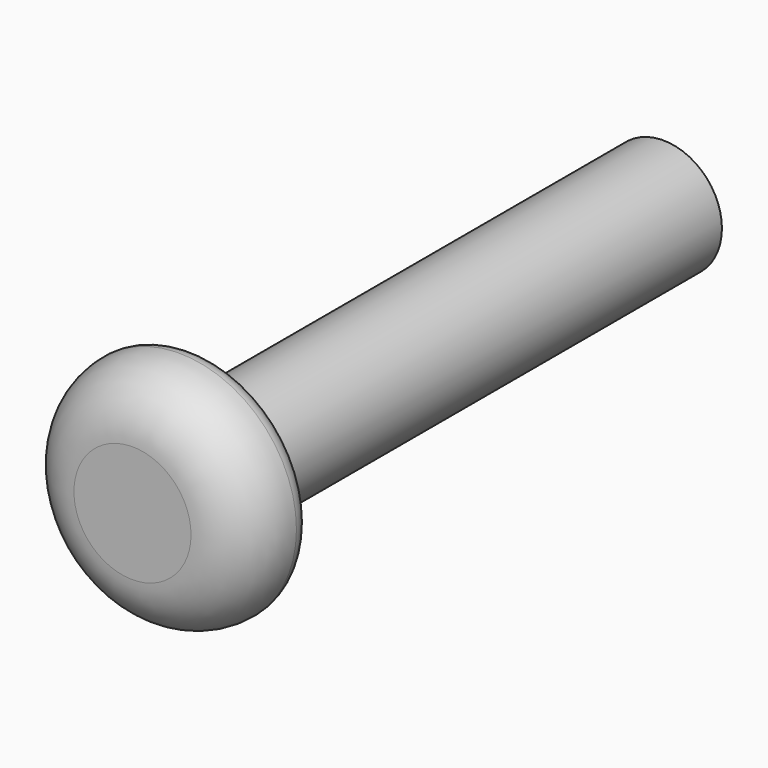
from build123d import *

# Parameters (mm, degrees)
F0_R     = 1.5
F1_DEPTH = 15
F2_R     = 3
F3_DEPTH = 2
F4_R     = 1.5
F5_R     = 0.49999


# Not quite as in the source:
# - a fillet or chamfer is up to 0.001 mm smaller than in the source, because OpenCascade refuses the exact size


with BuildPart() as f1:
    # F0 (on Front) → F1 (new body)
    with BuildSketch(Plane.XZ):
        Circle(F0_R)
    extrude(amount=-F1_DEPTH)

    # F2 (on face) → F3 (join)
    with BuildSketch(Plane.XZ):
        Circle(F2_R)
    extrude(amount=F3_DEPTH)

    # F4
    f4_edges = [f1.edges().sort_by_distance(p)[0] for p in [
        (-3, -2, 0),
    ]]
    fillet(f4_edges, radius=F4_R)

    # F5 (radius 0.5 in the source; OpenCascade refuses exactly that, so slightly less here)
    f5_edges = [f1.edges().sort_by_distance(p)[0] for p in [
        (-3, 0, 0),
    ]]
    fillet(f5_edges, radius=F5_R)


solid = f1.part
